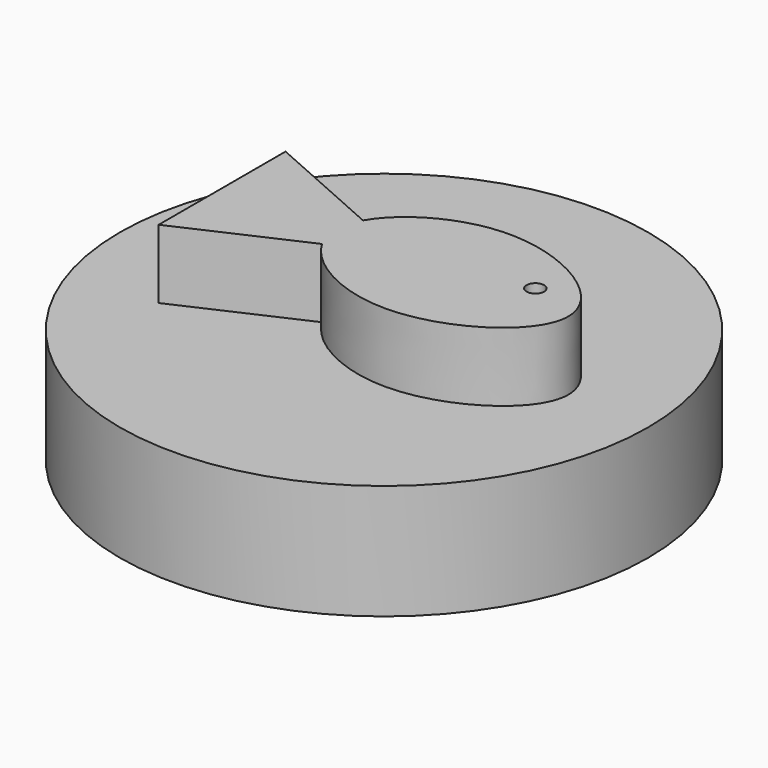
from build123d import *

# Parameters (mm, degrees)
F0_R     = 11.5
F1_DEPTH = 5
F3_DEPTH = 3
F4_R     = 0.3838948085
F5_DEPTH = 2


with BuildPart() as f1:
    # F0 (on Top) → F1 (new body)
    with BuildSketch(Plane.XY):
        with Locations((-31.1644673347, 23.6595552415)):
            Circle(F0_R)
    extrude(amount=F1_DEPTH)

    # F2 (on face) → F3 (join)
    with BuildSketch(Plane.XY.offset(5)):
        with BuildLine():
            add(Edge.make_bspline(
                [(-33.1539588035, 22.7823868875), (-33.3507914741, 23.1327616424), (-33.4622053799, 23.4998701067), (-33.4669202566, 23.8672532141)],
                knots=[0.9471889438, 0.9471889438, 0.9471889438, 0.9471889438, 1, 1, 1, 1], degree=3))
            add(Edge.make_bspline(
                [(-33.4669202566, 23.8672532141), (-33.47186302, 24.2523932514), (-33.3595432056, 24.6378351224), (-33.1539588035, 25.0042262209)],
                knots=[0, 0, 0, 0, 0.0553636021, 0.0553636021, 0.0553636021, 0.0553636021], degree=3))
            Line((-33.1539588035, 25.0042262209), (-38.3802689612, 27.3198802024))
            Line((-38.3802689612, 27.3198802024), (-38.3802689612, 20.4146262258))
            Line((-38.3802689612, 20.4146262258), (-33.1539588035, 22.7823868875))
        make_face()
        with BuildLine():
            add(Edge.make_bspline(
                [(-33.4669202566, 23.8672532141), (-33.47186302, 24.2523932514), (-33.3595432056, 24.6378351224), (-33.1539588035, 25.0042262209)],
                knots=[0, 0, 0, 0, 0.0553636021, 0.0553636021, 0.0553636021, 0.0553636021], degree=3))
            add(Edge.make_bspline(
                [(-33.1539588035, 22.7823868875), (-33.3507914741, 23.1327616424), (-33.4622053799, 23.4998701067), (-33.4669202566, 23.8672532141)],
                knots=[0.9471889438, 0.9471889438, 0.9471889438, 0.9471889438, 1, 1, 1, 1], degree=3))
            add(Edge.make_bspline(
                [(-33.1539588035, 25.0042262209), (-32.4560794327, 26.2479820054), (-28.2623769018, 28.6711404266), (-20.4801214372, 23.8919640928), (-28.1163432289, 19.0510090022), (-32.4328761402, 21.498813583), (-33.1539588035, 22.7823868875)],
                knots=[0.0553636021, 0.0553636021, 0.0553636021, 0.0553636021, 0.243301575, 0.499995332, 0.7537193486, 0.9471889438, 0.9471889438, 0.9471889438, 0.9471889438], degree=3))
        make_face()
    extrude(amount=F3_DEPTH)

    # F4 (on face) → F5 (cut)
    with BuildSketch(Plane.XY.offset(8)):
        with Locations((-25.4533700645, 24.7579738498)):
            Circle(F4_R)
    extrude(amount=-F5_DEPTH, mode=Mode.SUBTRACT)


solid = f1.part
